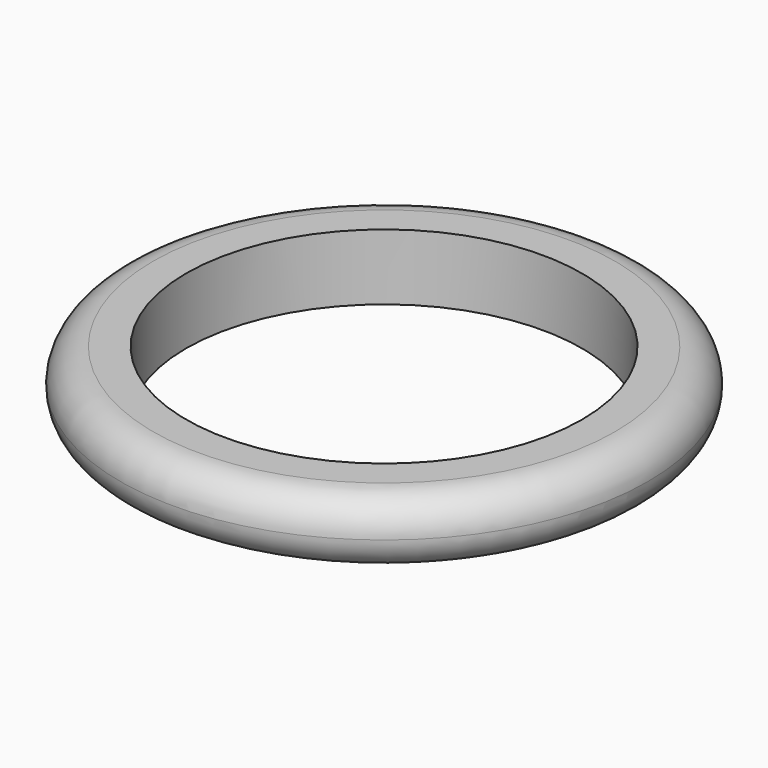
from build123d import *

# Parameters (mm, degrees)
F0_R     = 12.7
F0_R_2   = 9.525
F1_DEPTH = 3.175
F2_R     = 1.58749


# Not quite as in the source:
# - a fillet or chamfer is up to 0.001 mm smaller than in the source, because OpenCascade refuses the exact size


with BuildPart() as f1:
    # F0 (on Top) → F1 (new body)
    with BuildSketch(Plane.XY):
        Circle(F0_R)
        Circle(F0_R_2, mode=Mode.SUBTRACT)
    extrude(amount=F1_DEPTH)

    # F2 (radius 1.5875 in the source; OpenCascade refuses exactly that, so slightly less here)
    f2_edges = [f1.edges().sort_by_distance(p)[0] for p in [
        (-12.7, 0, 0),
        (-12.7, 0, 3.175),
    ]]
    fillet(f2_edges, radius=F2_R)


solid = f1.part
